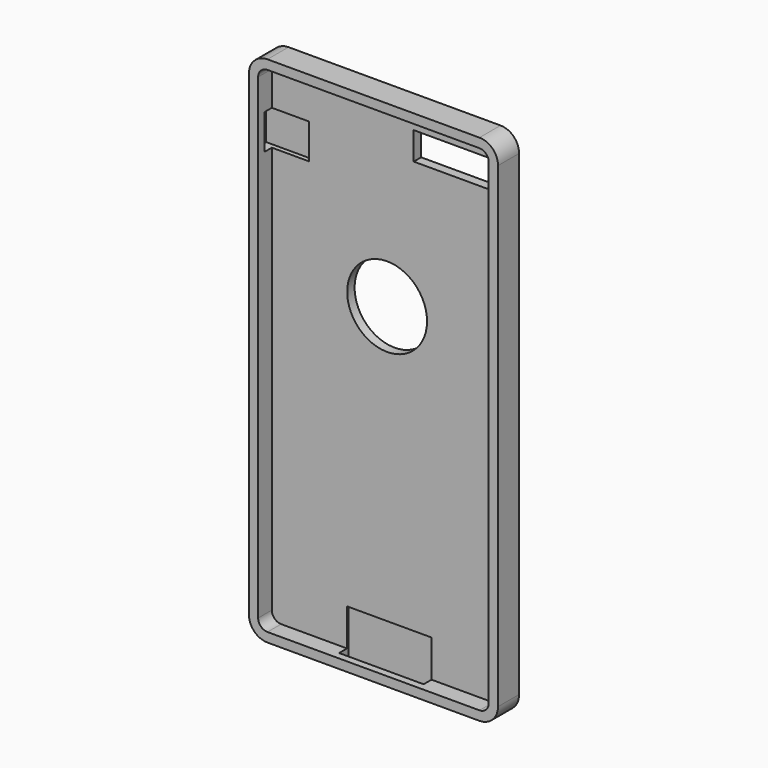
from build123d import *

# Parameters (mm, degrees)
F0_W      = 67.1
F0_H      = 138.3
F1_DEPTH  = 3.55
F2_R      = 5
F3_T      = -2.5
F4_W      = 20.0819657184
F4_H      = 7.4590183794
F5_DEPTH  = 12.5
F7_R      = 10.7534144168
F8_DEPTH  = 12.5
F6_W      = 22.7594478056
F6_H      = 3.1675179489
F9_DEPTH  = 12.5
F10_W     = 3.7042096956
F10_H     = 9.4521231949
F11_DEPTH = 12.5


with BuildPart() as f1:
    # F0 (on Front) → F1 (new body, symmetric)
    with BuildSketch(Plane.XZ):
        with Locations((0, -3.435843619)):
            Rectangle(F0_W, F0_H)
    extrude(amount=F1_DEPTH, both=True)

    # F2
    f2_edges = [f1.edges().sort_by_distance(p)[0] for p in [
        (33.55, 0, 65.714156),
        (33.55, 0, -72.585844),
        (-33.55, 0, -72.585844),
        (-33.55, 0, 65.714156),
    ]]
    fillet(f2_edges, radius=F2_R)

    # F3
    f3_openings = [f1.faces().sort_by_distance(p)[0] for p in [
        (0, -3.55, -3.435844),
    ]]
    offset(amount=F3_T, openings=f3_openings)

    # F4 (on face) → F5 (cut, symmetric)
    with BuildSketch(Plane.XZ.offset(-1.05)):
        with Locations((17.2131143045, 54.9385268241)):
            Rectangle(F4_W, F4_H)
    extrude(amount=F5_DEPTH, both=True, mode=Mode.SUBTRACT)

    # F7 (on face) → F8 (cut, symmetric)
    with BuildSketch(Plane.XZ.offset(-1.05)):
        with Locations((0, 14.4877051935)):
            Circle(F7_R)
    extrude(amount=F8_DEPTH, both=True, mode=Mode.SUBTRACT)

    # F6 (on face) → F9 (cut, symmetric)
    with BuildSketch(Plane(origin=(0, 0, -72.585843619), x_dir=(1, 0, 0), z_dir=(0, 0, -1))):
        with Locations((0.5839481018, 0.0267331488)):
            Rectangle(F6_W, F6_H)
    extrude(amount=F9_DEPTH, both=True, mode=Mode.SUBTRACT)

    # F10 (on face) → F11 (cut, symmetric)
    with BuildSketch(Plane(origin=(-33.55, 0, 0), x_dir=(0, -1, 0), z_dir=(-1, 0, 0))):
        with Locations((-0.4275311367, 46.8149799854)):
            Rectangle(F10_W, F10_H)
    extrude(amount=F11_DEPTH, both=True, mode=Mode.SUBTRACT)


solid = f1.part
